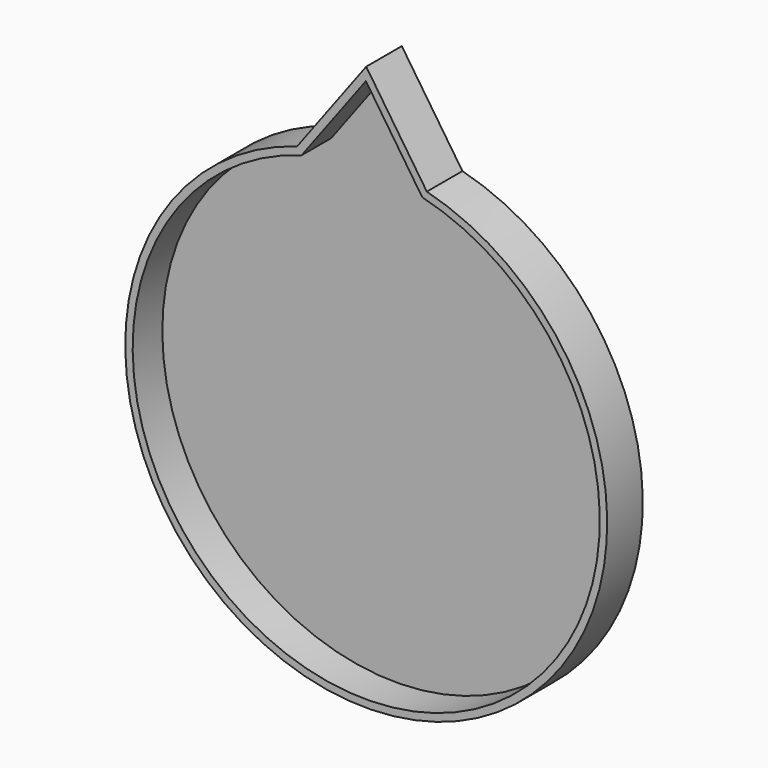
from build123d import *

# Parameters (mm, degrees)
F1_DEPTH = 12
F2_T     = -2


with BuildPart() as f1:
    # F0 (on Front) → F1 (new body)
    with BuildSketch(Plane.XZ):
        with BuildLine():
            Line((0, 87.2677220979), (-18.6475409836, 62.2677220979))
            ThreePointArc((-18.6475409836, 62.2677220979), (1.1915533371, -64.9890775488), (16.3524590164, 62.909435573))
            Line((16.3524590164, 62.909435573), (0, 87.2677220979))
        make_face()
    extrude(amount=F1_DEPTH)

    # F2
    f2_openings = [f1.faces().sort_by_distance(p)[0] for p in [
        (-0.019386, -12, 1.977046),
    ]]
    offset(amount=F2_T, openings=f2_openings, kind=Kind.INTERSECTION)


solid = f1.part
